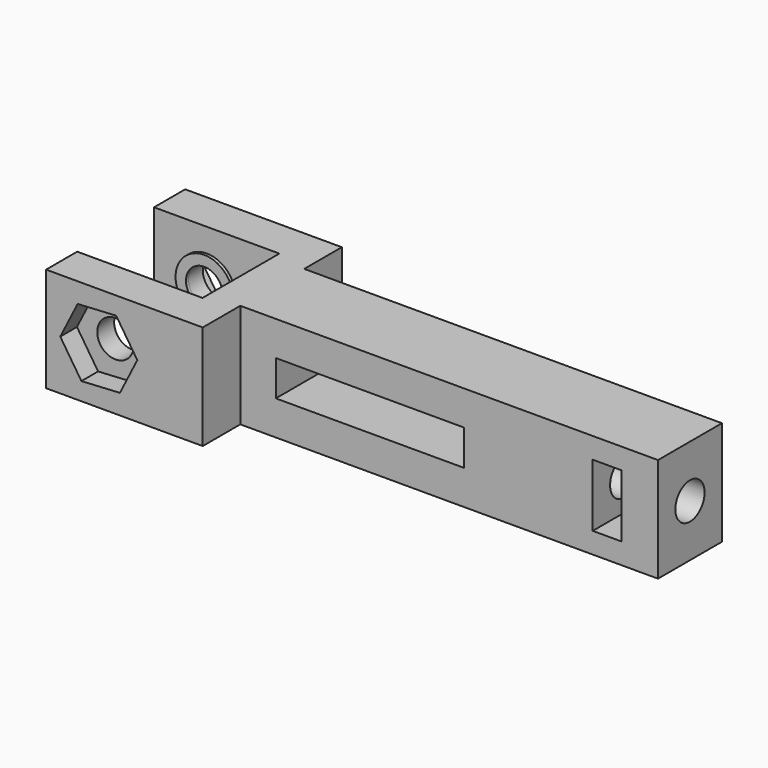
from build123d import *

# Parameters (mm, degrees)
F0_W      = 40
F0_H      = 3.825
F1_DEPTH  = 10
F2_R      = 1.75
F3_DEPTH  = 16.651
F4_W      = 18
F4_H      = 3.4
F4_W_2    = 2.75
F4_H_2    = 6
F5_DEPTH  = 12.151
F6_R      = 1.75
F7_DEPTH  = 15
F10_DEPTH = 2
F11_W     = 17.65
F11_H     = 60
F12_DEPTH = 8
F13_R     = 1.75
F14_DEPTH = 70.001
F15_R     = 2.75
F15_R_2   = 1.75
F16_DEPTH = 0.3
F17_R     = 1.75
F18_DEPTH = 2
F19_R     = 3.75
F20_DEPTH = 1


# Not quite as in the source:
# - a pattern or mirror of a feature is missing from the dataset's text; its kind, count and spacing are read off the source's solid


with BuildPart() as f1:
    # F0 (on Top) → F1 (new body)
    with BuildSketch(Plane.XY):
        Polygon((0, -3.825), (0, 0), (-3, 0), (-3, -4.6), (-15, -4.6), (-15, -8.325), (0, -8.325), align=None)
        Polygon((-3, 0), (0, 0), (0, 3.825), (0, 8.325), (-15, 8.325), (-15, 4.6), (-3, 4.6), align=None)
        with Locations((20, 1.9125)):
            Rectangle(F0_W, F0_H)
        with Locations((20, -1.9125)):
            Rectangle(F0_W, F0_H)
    extrude(amount=F1_DEPTH)

    # F2 (on face) → F3 (cut, through all)
    with BuildSketch(Plane.XZ.offset(8.325)):
        with Locations((-9.9527407438, 5)):
            Circle(F2_R)
    extrude(amount=-F3_DEPTH, mode=Mode.SUBTRACT)

    # F4 (on face) → F5 (cut, through all)
    with BuildSketch(Plane.XZ.offset(3.825)):
        with Locations((12.4002694301, 5)):
            Rectangle(F4_W, F4_H)
        with Locations((35.125, 5)):
            Rectangle(F4_W_2, F4_H_2)
    extrude(amount=-F5_DEPTH, mode=Mode.SUBTRACT)

    # F6 (on face) → F7 (cut)
    with BuildSketch(Plane.YZ.offset(40)):
        with Locations((0, 5)):
            Circle(F6_R)
    extrude(amount=-F7_DEPTH, mode=Mode.SUBTRACT)

    # F15 (on face) → F16 (join)
    with BuildSketch(Plane.XZ.offset(-4.6)):
        with Locations((-9.9527407438, 5)):
            Circle(F15_R)
        with Locations((-9.9527407438, 5)):
            Circle(F15_R_2, mode=Mode.SUBTRACT)
    f16 = extrude(amount=F16_DEPTH)

    # F16_copies: F16 across plane
    add(f16.mirror(Plane(origin=(0, 0, 0), x_dir=(0, 0, -1), z_dir=(0, -1, 0))))

    # F17 (on face) → F18 (cut)
    with BuildSketch(Plane.XZ.offset(8.325)):
        Polygon((-7.9284293953, 1.9088033227), (-6.2635302189, 5.2075067143), (-8.2878415673, 8.2987033916), (-11.9770520922, 8.0911966773), (-13.6419512686, 4.7924932857), (-11.6176399202, 1.7012966084), align=None)
        with Locations((-9.9527407438, 5)):
            Circle(F17_R, mode=Mode.SUBTRACT)
    f18 = extrude(amount=-F18_DEPTH, mode=Mode.SUBTRACT)

    # F18_copies: F18 across plane
    add(f18.mirror(Plane.ZX), mode=Mode.SUBTRACT)


with BuildPart() as f10:
    # F9 (on offset) → F10 (new body)
    with BuildSketch(Plane.YZ.offset(45)):
        Polygon((3.825, 0), (3.825, 10), (3.825, 19.8484882712), (-3.825, 19.8484882712), (-3.825, 10), (-3.825, 0), (-3.825, -10.1515117288), (3.825, -10.1515117288), align=None)
    extrude(amount=F10_DEPTH)

    # F11 (on face) → F12 (join)
    with BuildSketch(Plane.YZ.offset(47)):
        with Locations((0, 4.8484882712)):
            Rectangle(F11_W, F11_H)
    extrude(amount=F12_DEPTH)

    # F13 (on face) → F14 (cut, through all)
    with BuildSketch(Plane.YZ.offset(55)):
        with Locations((0, 5)):
            Circle(F13_R)
    extrude(amount=-F14_DEPTH, mode=Mode.SUBTRACT)

    # F19 (on face) → F20 (join)
    with BuildSketch(Plane(origin=(47, 0, 0), x_dir=(0, -1, 0), z_dir=(-1, 0, 0))):
        with Locations((0, -18)):
            Circle(F19_R)
        with Locations((0, 28)):
            Circle(F19_R)
    extrude(amount=F20_DEPTH)


solid = f1.part
